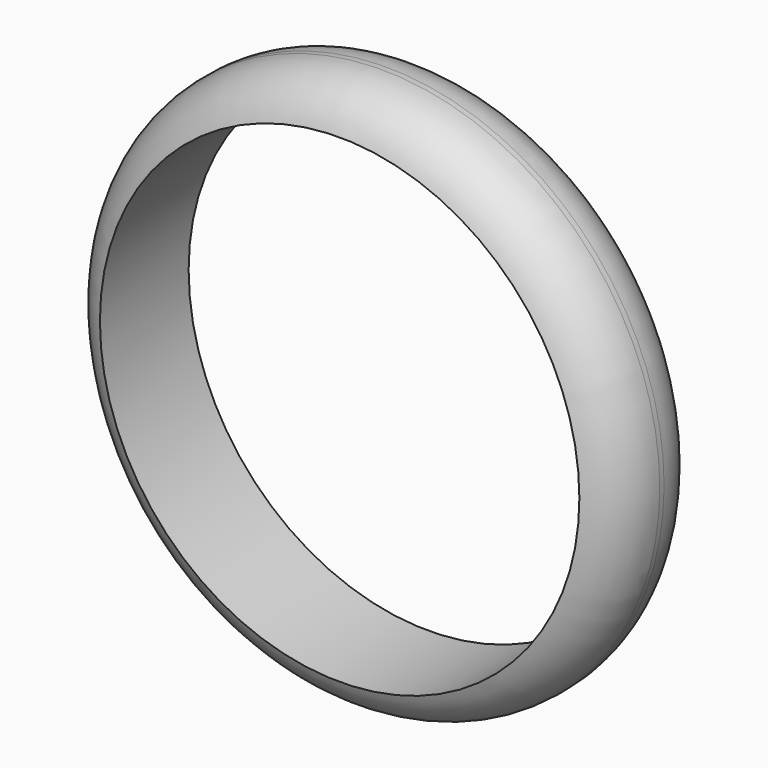
from build123d import *

# Parameters (mm, degrees)
F0_R     = 12.5312471482
F1_DEPTH = 2.5
F2_R     = 10.8098139949
F3_DEPTH = 75.98543


# Not quite as in the source:
# - a fillet or chamfer that OpenCascade refuses, or shapes differently, is made with other operations: its cross-section is extruded or revolved along the edge and cut away or added


with BuildPart() as f1:
    # F0 (on Front) → F1 (new body, symmetric)
    with BuildSketch(Plane.XZ):
        Circle(F0_R)
    extrude(amount=F1_DEPTH, both=True)

    # F2 (on face) → F3 (cut)
    with BuildSketch(Plane.XZ.offset(2.5)):
        Circle(F2_R)
    extrude(amount=-F3_DEPTH, mode=Mode.SUBTRACT)

    # F4: fillet of radius 2.5 on 1 edges, made by hand

    # F4_s1 → F4_t2 (revolve, cut)
    with BuildSketch(Plane.XY):
        with BuildLine():
            ThreePointArc((12.5312471482, -0.1243245876), (12.055650408, -1.5912231668), (10.8098139949, -2.5))
            Line((10.8098139949, -2.5), (12.5312471482, -2.5))
            Line((12.5312471482, -2.5), (12.5312471482, -0.1243245876))
        make_face()
    revolve(axis=Axis((0, -2.5, 0), (0, -1, 0)), mode=Mode.SUBTRACT)

    # F5: fillet of radius 2.5 on 1 edges, made by hand

    # F5_s1 → F5_t2 (revolve, cut)
    with BuildSketch(Plane.XY):
        with BuildLine():
            ThreePointArc((12.5312471482, 0.1243245876), (12.055650408, 1.5912231668), (10.8098139949, 2.5))
            Line((10.8098139949, 2.5), (12.5312471482, 2.5))
            Line((12.5312471482, 2.5), (12.5312471482, 0.1243245876))
        make_face()
    revolve(axis=Axis((0, 2.5, 0), (0, -1, 0)), mode=Mode.SUBTRACT)


solid = f1.part
